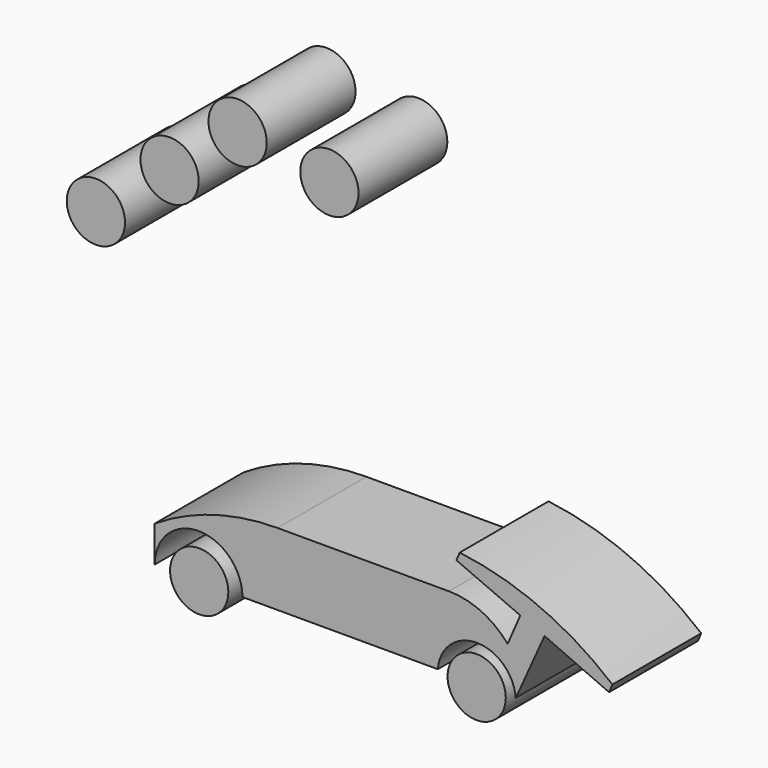
from build123d import *

# Parameters (mm, degrees)
F0_R     = 6.6651774255
F1_DEPTH = 25.4
F2_DEPTH = 25.4


# Not quite as in the source:
# - a feature names something its author has since deleted; it is built from what else it names


with BuildPart() as f1:
    # F0 (on Front) → F1 (new body)
    with BuildSketch(Plane.XZ):
        with Locations((63.0971782387, -32.2904203791)):
            Circle(F0_R)
    extrude(amount=F1_DEPTH)

    # F0 (on Front) → F2 (join)
    with BuildSketch(Plane.XZ):
        with Locations((63.0971782387, -32.2904203791)):
            Circle(F0_R)
    extrude(amount=F2_DEPTH)


with BuildPart() as f2:
    # F0 (on Front) → F2, piece 2 (new body)
    with BuildSketch(Plane.XZ):
        with Locations((79.9629938861, -18.4615177807)):
            Circle(F0_R)
    extrude(amount=F2_DEPTH)


with BuildPart() as f2b:
    # F0 (on Front) → F2, piece 3 (new body)
    with BuildSketch(Plane.XZ):
        with Locations((95.5259158782, -5.706744201)):
            Circle(F0_R)
    extrude(amount=F2_DEPTH)


with BuildPart() as f2c:
    # F0 (on Front) → F2, piece 4 (new body)
    with BuildSketch(Plane.XZ):
        with Locations((116.5277564155, -8.9942043108)):
            Circle(F0_R)
    extrude(amount=F2_DEPTH)


with BuildPart() as f2d:
    # F0 (on Front) → F2, piece 5 (new body)
    with BuildSketch(Plane.XZ):
        with BuildLine():
            ThreePointArc((157.310231805, -88.7043293319), (151.2945416105, -84.1069008982), (143.901631238, -82.4729630341))
            Line((143.901631238, -82.4729630341), (104.6853437268, -82.4729630341))
            ThreePointArc((104.6853437268, -82.4729630341), (90.0244825693, -84.5811974693), (76.5517114458, -90.7350532171))
            Line((76.5517114458, -90.7350532171), (76.5517114458, -98.9971434001))
            ThreePointArc((76.5517114458, -98.9971434001), (86.591364621, -88.957490225), (96.6310177961, -98.9971434001))
            Line((96.6310177961, -98.9971434001), (141.3318150355, -98.9971434001))
            ThreePointArc((141.3318150355, -98.9971434001), (150.2522141557, -90.7635242584), (159.1726132759, -98.9971434001))
            Line((159.1726132759, -98.9971434001), (165.7533920403, -84.3646685002))
            Line((165.7533920403, -84.3646685002), (160.2166072323, -82.0221779593))
            Line((160.2166072323, -82.0221779593), (157.310231805, -88.7043293319))
        make_face()
        with BuildLine():
            Line((145.5935956957, -75.6619566722), (160.2166072323, -82.0221779593))
            Line((160.2166072323, -82.0221779593), (165.7533920403, -84.3646685002))
            Line((165.7533920403, -84.3646685002), (180.5155317609, -90.8968567243))
            Line((180.5155317609, -90.8968567243), (181.2792439876, -89.0917223253))
            ThreePointArc((181.2792439876, -89.0917223253), (164.9152343167, -78.9580413658), (146.3532217869, -73.8664803927))
            Line((146.3532217869, -73.8664803927), (145.5935956957, -75.6619566722))
        make_face()
    extrude(amount=F2_DEPTH)


with BuildPart() as f2e:
    # F0 (on Front) → F2, piece 6 (new body)
    with BuildSketch(Plane.XZ):
        with Locations((86.7331768035, -99.0469055689)):
            Circle(F0_R)
    extrude(amount=F2_DEPTH)


with BuildPart() as f2f:
    # F0 (on Front) → F2, piece 7 (new body)
    with BuildSketch(Plane.XZ):
        with Locations((150.2222788557, -99.7178808889)):
            Circle(F0_R)
    extrude(amount=F2_DEPTH)


solid = Compound([f1.part, f2.part, f2b.part, f2c.part, f2d.part, f2e.part, f2f.part])
